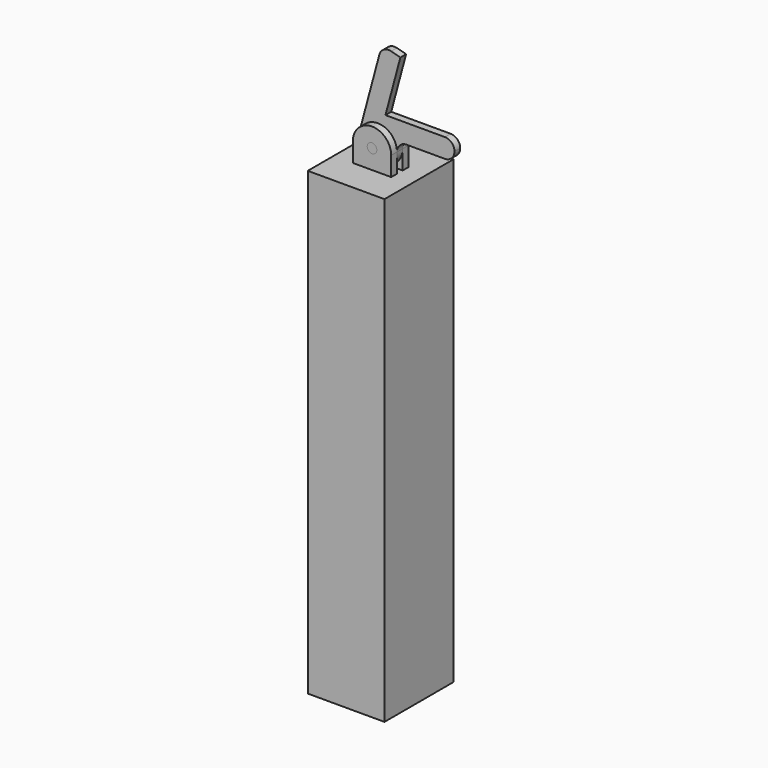
from build123d import *

# Parameters (mm, degrees)
F0_R          = 3.175
F1_DEPTH      = 4.7625
F3_DEPTH      = 9.525
F3_DEPTH_BACK = 4.7625
F6_DEPTH      = 2.38125
F7_W          = 50.8
F7_H          = 57.15
F7_W_2        = 25.4
F7_H_2        = 4.7625
F8_DEPTH      = 304.8


# Not quite as in the source:
# - a feature names something its author has since deleted; it is built from what else it names


with BuildPart() as f1:
    # F0 (on Front) → F1 (new body)
    with BuildSketch(Plane.XZ):
        with BuildLine():
            Line((12.7, -12.7), (12.7, 0))
            ThreePointArc((12.7, 0), (0, 12.7), (-12.7, 0))
            Line((-12.7, 0), (-12.7, -12.7))
            Line((-12.7, -12.7), (0, -12.7))
            Line((0, -12.7), (12.7, -12.7))
        make_face()
        Circle(F0_R, mode=Mode.SUBTRACT)
    extrude(amount=F1_DEPTH)


with BuildPart() as f2_1:
    # F2: copy of F1
    add(f1.part.moved(Location((0, 9.525, 0))))


with BuildPart() as f3:
    # F0 (on Front) → F3 (new body, two sides)
    with BuildSketch(Plane.XZ) as f3_sk:
        Circle(F0_R)
    extrude(amount=-F3_DEPTH)
    extrude(f3_sk.sketch, amount=F3_DEPTH_BACK)


with BuildPart() as f6:
    # F5 (on offset) → F6 (new body, symmetric)
    with BuildSketch(Plane.XZ.offset(-2.38125)):
        with BuildLine():
            ThreePointArc((50.8, 12.7), (48.9401280605, 17.1901280605), (44.45, 19.05))
            Line((44.45, 19.05), (5.1044321158, 19.05))
            Line((5.1044321158, 19.05), (14.9654377342, 55.8517739816))
            Line((14.9654377342, 55.8517739816), (8.8318087373, 57.495274918))
            ThreePointArc((8.8318087373, 57.495274918), (4.0133078009, 56.8609072351), (1.0546788039, 53.0051468575))
            Line((1.0546788039, 53.0051468575), (-12.2672579939, 3.2870018728))
            ThreePointArc((-12.2672579939, 3.2870018728), (-1.6576826412, -12.5913497394), (12.7, 0))
            ThreePointArc((12.7, 0), (14.5598719395, 4.4901280605), (19.05, 6.35))
            Line((19.05, 6.35), (44.45, 6.35))
            ThreePointArc((44.45, 6.35), (48.9401280605, 8.2098719395), (50.8, 12.7))
        make_face()
    extrude(amount=F6_DEPTH, both=True)


with BuildPart() as f8:
    # F7 (on face) → F8 (new body)
    with BuildSketch(Plane(origin=(0, 0, -12.7), x_dir=(1, 0, 0), z_dir=(0, 0, -1))):
        with Locations((0, -2.38125)):
            Rectangle(F7_W, F7_H)
        with Locations((0, 2.38125)):
            Rectangle(F7_W_2, F7_H_2, mode=Mode.SUBTRACT)
        with Locations((0, 2.38125)):
            Rectangle(F7_W_2, F7_H_2)
    extrude(amount=F8_DEPTH)


solid = Compound([f1.part, f2_1.part, f3.part, f6.part, f8.part])
